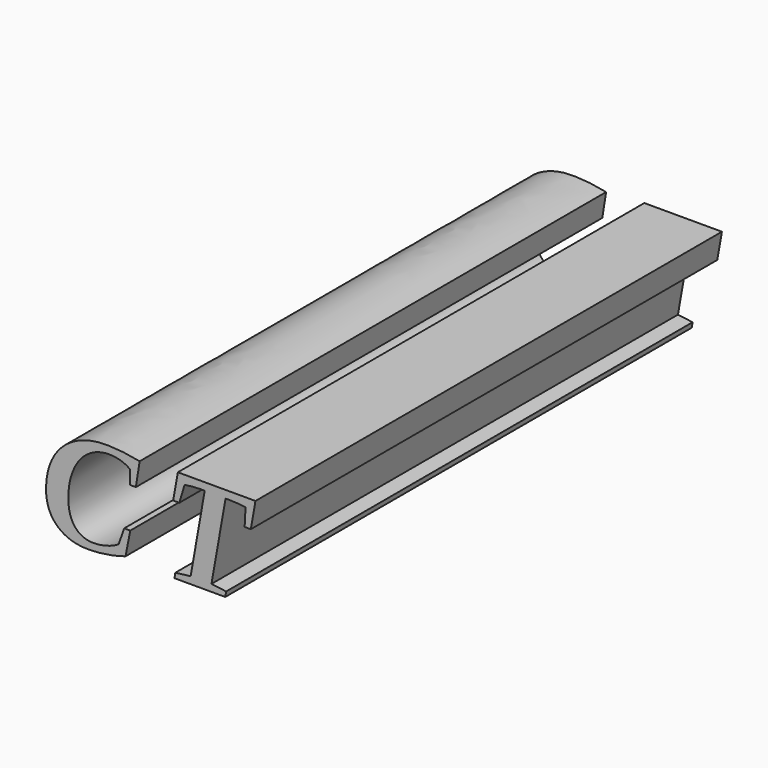
from build123d import *

# Parameters (mm, degrees)
F0_TEXT_SIZE   = 31.75
F0_TEXT_SIZE_2 = 31.3892039767
F1_DEPTH       = 127


# Not quite as in the source:
# - Text() gives the source's letters only with a copy of the font that has no kerning and outlines rounded to 1/6400 em; it was checked with that copy


with BuildPart() as f1:
    # F0 (on Front) → F1 (new body)
    with BuildSketch(Plane.XZ):
        with Locations((-20.2298000055, -4.1238920315)):
            Text('C', F0_TEXT_SIZE, font='Tinos', font_style=FontStyle.BOLDITALIC, text_align=(TextAlign.LEFT, TextAlign.BOTTOM))
        with Locations((6.2670164637, -3.8641188947)):
            Text('T', F0_TEXT_SIZE_2, font='Tinos', font_style=FontStyle.BOLDITALIC, text_align=(TextAlign.LEFT, TextAlign.BOTTOM))
    extrude(amount=F1_DEPTH)


solid = f1.part
